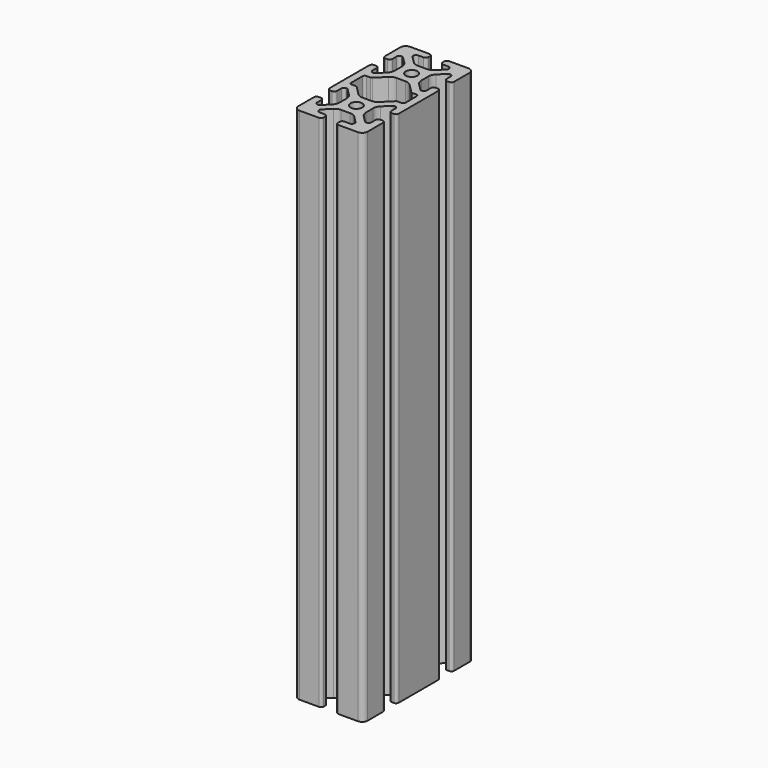
from build123d import *

# Parameters (mm, degrees)
F1_R     = 3.4
F2_DEPTH = 300


# Not quite as in the source:
# - ends of sketch curves that miss each other by under 0.0002 mm in the source are joined


with BuildPart() as f2:
    # F1 (on Top) → F2 (new body)
    with BuildSketch(Plane.XY):
        with BuildLine():
            Line((5.690449, -40), (16.83, -40))
            ThreePointArc((16.83, -40), (19.0715284964, -39.0715284964), (20, -36.83))
            Line((20, -36.83), (20, -25.690449))
            ThreePointArc((20, -25.690449), (19.5401576465, -24.5802913535), (18.43, -24.120449))
            Line((18.43, -24.120449), (17.25, -24.120449))
            ThreePointArc((17.25, -24.120449), (16.1398423535, -24.5802913535), (15.68, -25.690449))
            Line((15.68, -25.690449), (15.68, -28.715399))
            ThreePointArc((15.68, -28.715399), (15.2201576465, -29.8255566465), (14.11, -30.285399))
            Line((14.11, -30.285399), (13.654903, -30.2854))
            ThreePointArc((13.654903, -30.2854), (13.364063918, -30.22754758), (13.1175023463, -30.0628006537))
            Line((13.1175023463, -30.0628006537), (9.109794, -26.055093))
            ThreePointArc((9.109794, -26.055093), (8.0552918962, -24.4769190736), (7.685, -22.615336))
            Line((7.685, -22.615336), (7.685, -17.384664))
            ThreePointArc((7.685, -17.384664), (8.0552918962, -15.5230809264), (9.1097940005, -13.9449070005))
            Line((9.1097940005, -13.9449070005), (13.117502, -9.937199))
            ThreePointArc((13.117502, -9.937199), (13.364063918, -9.77245242), (13.654903, -9.714601))
            Line((13.654903, -9.714601), (14.11, -9.7146))
            ThreePointArc((14.11, -9.7146), (15.2201576465, -10.1744433535), (15.68, -11.284601))
            Line((15.68, -11.284601), (15.68, -14.309551))
            ThreePointArc((15.68, -14.309551), (16.1398423535, -15.4197086465), (17.25, -15.879551))
            Line((17.25, -15.879551), (18.43, -15.879551))
            ThreePointArc((18.43, -15.879551), (19.5401576465, -15.4197086465), (20, -14.309551))
            Line((20, -14.309551), (20, 14.309551))
            ThreePointArc((20, 14.309551), (19.5401576465, 15.4197086465), (18.43, 15.879551))
            Line((18.43, 15.879551), (17.25, 15.879551))
            ThreePointArc((17.25, 15.879551), (16.1398423535, 15.4197086465), (15.68, 14.309551))
            Line((15.68, 14.309551), (15.68, 11.2846))
            ThreePointArc((15.68, 11.2846), (15.2201576465, 10.1744423535), (14.11, 9.7146))
            Line((14.11, 9.7146), (13.654903, 9.7146))
            ThreePointArc((13.654903, 9.7146), (13.364063918, 9.77245242), (13.1175023463, 9.9371993463))
            Line((13.1175023463, 9.9371993463), (9.109794, 13.944907))
            ThreePointArc((9.109794, 13.944907), (8.0552918962, 15.5230809264), (7.685, 17.384664))
            Line((7.685, 17.384664), (7.685, 22.615336))
            ThreePointArc((7.685, 22.615336), (8.0552918962, 24.4769190736), (9.1097940005, 26.0550929995))
            Line((9.1097940005, 26.0550929995), (13.117502, 30.062801))
            ThreePointArc((13.117502, 30.062801), (13.364063918, 30.22754758), (13.654903, 30.285399))
            Line((13.654903, 30.285399), (14.11, 30.2854))
            ThreePointArc((14.11, 30.2854), (15.2201576465, 29.8255576465), (15.68, 28.7154))
            Line((15.68, 28.7154), (15.68, 25.690449))
            ThreePointArc((15.68, 25.690449), (16.1398423535, 24.5802913535), (17.25, 24.120449))
            Line((17.25, 24.120449), (18.43, 24.120449))
            ThreePointArc((18.43, 24.120449), (19.5401576465, 24.5802913535), (20, 25.690449))
            Line((20, 25.690449), (20, 36.83))
            ThreePointArc((20, 36.83), (19.0715284964, 39.0715284964), (16.83, 40))
            Line((16.83, 40), (5.690449, 40))
            ThreePointArc((5.690449, 40), (4.5802913535, 39.5401576465), (4.120449, 38.43))
            Line((4.120449, 38.43), (4.120449, 37.25))
            ThreePointArc((4.120449, 37.25), (4.5802913535, 36.1398423535), (5.690449, 35.68))
            Line((5.690449, 35.68), (8.7154, 35.68))
            ThreePointArc((8.7154, 35.68), (9.8255576465, 35.2201576465), (10.2854, 34.11))
            Line((10.2854, 34.11), (10.2854, 33.654903))
            ThreePointArc((10.2854, 33.654903), (10.2275484447, 33.3640635914), (10.0628011537, 33.1175018463))
            Line((10.0628011537, 33.1175018463), (6.055093, 29.109794))
            ThreePointArc((6.055093, 29.109794), (4.4769190736, 28.0552918962), (2.615336, 27.685))
            Line((2.615336, 27.685), (-2.615336, 27.685))
            ThreePointArc((-2.615336, 27.685), (-4.4769190736, 28.0552918962), (-6.0550929995, 29.1097940005))
            Line((-6.0550929995, 29.1097940005), (-10.062801, 33.117502))
            ThreePointArc((-10.062801, 33.117502), (-10.22754758, 33.364063918), (-10.285399, 33.654903))
            Line((-10.285399, 33.654903), (-10.2854, 34.11))
            ThreePointArc((-10.2854, 34.11), (-9.8255576465, 35.2201576465), (-8.7154, 35.68))
            Line((-8.7154, 35.68), (-5.690449, 35.68))
            ThreePointArc((-5.690449, 35.68), (-4.5802913535, 36.1398423535), (-4.120449, 37.25))
            Line((-4.120449, 37.25), (-4.120449, 38.43))
            ThreePointArc((-4.120449, 38.43), (-4.5802913535, 39.5401576465), (-5.690449, 40))
            Line((-5.690449, 40), (-16.83, 40))
            ThreePointArc((-16.83, 40), (-19.0715284964, 39.0715284964), (-20, 36.83))
            Line((-20, 36.83), (-20, 25.690449))
            ThreePointArc((-20, 25.690449), (-19.5401576465, 24.5802913535), (-18.43, 24.120449))
            Line((-18.43, 24.120449), (-17.25, 24.120449))
            ThreePointArc((-17.25, 24.120449), (-16.1398423535, 24.5802913535), (-15.68, 25.690449))
            Line((-15.68, 25.690449), (-15.68, 28.7154))
            ThreePointArc((-15.68, 28.7154), (-15.2201576465, 29.8255576465), (-14.11, 30.2854))
            Line((-14.11, 30.2854), (-13.654903, 30.2854))
            ThreePointArc((-13.654903, 30.2854), (-13.3640635914, 30.2275484447), (-13.1175018463, 30.0628011537))
            Line((-13.1175018463, 30.0628011537), (-9.109794, 26.055093))
            ThreePointArc((-9.109794, 26.055093), (-8.0552918962, 24.4769190736), (-7.685, 22.615336))
            Line((-7.685, 22.615336), (-7.685, 17.384664))
            ThreePointArc((-7.685, 17.384664), (-8.0552918962, 15.5230809264), (-9.1097940005, 13.9449070005))
            Line((-9.1097940005, 13.9449070005), (-13.117502, 9.937199))
            ThreePointArc((-13.117502, 9.937199), (-13.364063918, 9.77245242), (-13.654903, 9.714601))
            Line((-13.654903, 9.714601), (-14.11, 9.7146))
            ThreePointArc((-14.11, 9.7146), (-15.2201576465, 10.1744423535), (-15.68, 11.2846))
            Line((-15.68, 11.2846), (-15.68, 14.309551))
            ThreePointArc((-15.68, 14.309551), (-16.1398423535, 15.4197086465), (-17.25, 15.879551))
            Line((-17.25, 15.879551), (-18.43, 15.879551))
            ThreePointArc((-18.43, 15.879551), (-19.5401576465, 15.4197086465), (-20, 14.309551))
            Line((-20, 14.309551), (-20, -14.309551))
            ThreePointArc((-20, -14.309551), (-19.5401576465, -15.4197086465), (-18.43, -15.879551))
            Line((-18.43, -15.879551), (-17.25, -15.879551))
            ThreePointArc((-17.25, -15.879551), (-16.1398423535, -15.4197086465), (-15.68, -14.309551))
            Line((-15.68, -14.309551), (-15.68, -11.284601))
            ThreePointArc((-15.68, -11.284601), (-15.2201576465, -10.1744433535), (-14.11, -9.714601))
            Line((-14.11, -9.714601), (-13.654903, -9.7146))
            ThreePointArc((-13.654903, -9.7146), (-13.364063918, -9.77245242), (-13.1175023463, -9.9371993463))
            Line((-13.1175023463, -9.9371993463), (-9.109794, -13.944907))
            ThreePointArc((-9.109794, -13.944907), (-8.0552918962, -15.5230809264), (-7.685, -17.384664))
            Line((-7.685, -17.384664), (-7.685, -22.615336))
            ThreePointArc((-7.685, -22.615336), (-8.0552918962, -24.4769190736), (-9.1097940005, -26.0550929995))
            Line((-9.1097940005, -26.0550929995), (-13.117502, -30.062801))
            ThreePointArc((-13.117502, -30.062801), (-13.364063918, -30.22754758), (-13.654903, -30.285399))
            Line((-13.654903, -30.285399), (-14.11, -30.2854))
            ThreePointArc((-14.11, -30.2854), (-15.2201576465, -29.8255566465), (-15.68, -28.715399))
            Line((-15.68, -28.715399), (-15.68, -25.690449))
            ThreePointArc((-15.68, -25.690449), (-16.1398423535, -24.5802913535), (-17.25, -24.120449))
            Line((-17.25, -24.120449), (-18.43, -24.120449))
            ThreePointArc((-18.43, -24.120449), (-19.5401576465, -24.5802913535), (-20, -25.690449))
            Line((-20, -25.690449), (-20, -36.83))
            ThreePointArc((-20, -36.83), (-19.0715284964, -39.0715284964), (-16.83, -40))
            Line((-16.83, -40), (-5.690449, -40))
            ThreePointArc((-5.690449, -40), (-4.5802913535, -39.5401576465), (-4.120449, -38.43))
            Line((-4.120449, -38.43), (-4.120449, -37.25))
            ThreePointArc((-4.120449, -37.25), (-4.5802913535, -36.1398423535), (-5.690449, -35.68))
            Line((-5.690449, -35.68), (-8.7154, -35.68))
            ThreePointArc((-8.7154, -35.68), (-9.8255576465, -35.2201576465), (-10.2854, -34.11))
            Line((-10.2854, -34.11), (-10.2854, -33.654903))
            ThreePointArc((-10.2854, -33.654903), (-10.2275484447, -33.3640635914), (-10.0628011537, -33.1175018463))
            Line((-10.0628011537, -33.1175018463), (-6.055093, -29.109794))
            ThreePointArc((-6.055093, -29.109794), (-4.4769190736, -28.0552918962), (-2.615336, -27.685))
            Line((-2.615336, -27.685), (2.615336, -27.685))
            ThreePointArc((2.615336, -27.685), (4.4769190736, -28.0552918962), (6.0550929995, -29.1097940005))
            Line((6.0550929995, -29.1097940005), (10.062801, -33.117502))
            ThreePointArc((10.062801, -33.117502), (10.22754758, -33.364063918), (10.285399, -33.654903))
            Line((10.285399, -33.654903), (10.2854, -34.11))
            ThreePointArc((10.2854, -34.11), (9.8255576465, -35.2201576465), (8.7154, -35.68))
            Line((8.7154, -35.68), (5.690449, -35.68))
            ThreePointArc((5.690449, -35.68), (4.5802913535, -36.1398423535), (4.120449, -37.25))
            Line((4.120449, -37.25), (4.120449, -38.43))
            ThreePointArc((4.120449, -38.43), (4.5802913535, -39.5401576465), (5.690449, -40))
        make_face()
        with Locations((0, -20)):
            Circle(F1_R, mode=Mode.SUBTRACT)
        with BuildLine():
            Line((15.68, 4.071352), (15.68, -4.071352))
            ThreePointArc((15.68, -4.071352), (15.3080256121, -4.9693776121), (14.41, -5.341352))
            Line((14.41, -5.341352), (12.129998, -5.341352))
            ThreePointArc((12.129998, -5.341352), (11.6439903675, -5.4380248584), (11.2319728879, -5.7133258879))
            Line((11.2319728879, -5.7133258879), (6.055093, -10.890206))
            ThreePointArc((6.055093, -10.890206), (4.4769190736, -11.9447081038), (2.615336, -12.315))
            Line((2.615336, -12.315), (-2.615336, -12.315))
            ThreePointArc((-2.615336, -12.315), (-4.4769190736, -11.9447081038), (-6.0550929995, -10.8902059995))
            Line((-6.0550929995, -10.8902059995), (-11.231973, -5.713326))
            ThreePointArc((-11.231973, -5.713326), (-11.6439903675, -5.4380248584), (-12.129998, -5.341352))
            Line((-12.129998, -5.341352), (-14.41, -5.341352))
            ThreePointArc((-14.41, -5.341352), (-15.3080256121, -4.9693776121), (-15.68, -4.071352))
            Line((-15.68, -4.071352), (-15.68, 4.071352))
            ThreePointArc((-15.68, 4.071352), (-15.3080256121, 4.9693776121), (-14.41, 5.341352))
            Line((-14.41, 5.341352), (-12.129998, 5.341352))
            ThreePointArc((-12.129998, 5.341352), (-11.6439903675, 5.4380248584), (-11.2319728879, 5.7133258879))
            Line((-11.2319728879, 5.7133258879), (-6.055093, 10.890206))
            ThreePointArc((-6.055093, 10.890206), (-4.4769190736, 11.9447081038), (-2.615336, 12.315))
            Line((-2.615336, 12.315), (2.615336, 12.315))
            ThreePointArc((2.615336, 12.315), (4.4769190736, 11.9447081038), (6.0550929995, 10.8902059995))
            Line((6.0550929995, 10.8902059995), (11.231973, 5.713326))
            ThreePointArc((11.231973, 5.713326), (11.6439903675, 5.4380248584), (12.129998, 5.341352))
            Line((12.129998, 5.341352), (14.41, 5.341352))
            ThreePointArc((14.41, 5.341352), (15.3080256121, 4.9693776121), (15.68, 4.071352))
        make_face(mode=Mode.SUBTRACT)
        with Locations((0, 20)):
            Circle(F1_R, mode=Mode.SUBTRACT)
    extrude(amount=F2_DEPTH)


solid = f2.part
